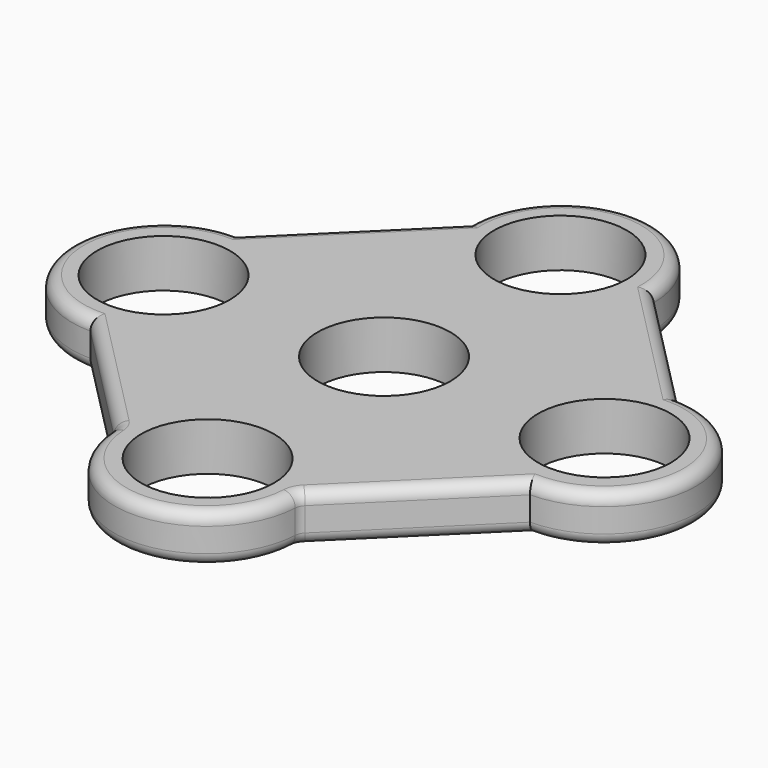
from build123d import *

# Parameters (mm, degrees)
F0_R     = 11.05
F1_DEPTH = 8
F2_R     = 2


with BuildPart() as f1:
    # F0 (on Top) → F1 (new body)
    with BuildSketch(Plane.XY):
        with BuildLine():
            Line((36.6952344775, 15.2133565883), (15.5011650662, 36.6952344775))
            ThreePointArc((15.5011650662, 36.6952344775), (0.1439042389, 52.0524953048), (-15.2133565883, 36.6952344775))
            Line((-15.2133565883, 36.6952344775), (-36.6952344775, 15.5011650662))
            ThreePointArc((-36.6952344775, 15.5011650662), (-52.0524953048, 0.1439042389), (-36.6952344775, -15.2133565883))
            Line((-36.6952344775, -15.2133565883), (-15.5011650662, -36.6952344775))
            ThreePointArc((-15.5011650662, -36.6952344775), (-0.1439042389, -52.0524953048), (15.2133565883, -36.6952344775))
            Line((15.2133565883, -36.6952344775), (36.6952344775, -15.5011650662))
            ThreePointArc((36.6952344775, -15.5011650662), (52.0524953048, -0.1439042389), (36.6952344775, 15.2133565883))
        make_face()
        with Locations((0, -36.6952344775)):
            Circle(F0_R, mode=Mode.SUBTRACT)
        with Locations((-36.6952344775, 0)):
            Circle(F0_R, mode=Mode.SUBTRACT)
        Circle(F0_R, mode=Mode.SUBTRACT)
        with Locations((0, 36.6952344775)):
            Circle(F0_R, mode=Mode.SUBTRACT)
        with Locations((36.6952344775, 0)):
            Circle(F0_R, mode=Mode.SUBTRACT)
    extrude(amount=F1_DEPTH)

    # F2
    f2_edges = [f1.edges().sort_by_distance(p)[0] for p in [
        (-25.954296, 26.0982, 8),
        (0.143904, 52.052495, 8),
        (26.0982, 25.954296, 8),
        (52.052495, -0.143904, 8),
        (25.954296, -26.0982, 8),
        (-0.143904, -52.052495, 8),
        (-26.0982, -25.954296, 8),
        (-52.052495, 0.143904, 8),
        (-15.501165, -36.695234, 4),
        (15.213357, -36.695234, 4),
        (-0.143904, -52.052495, 0),
        (25.954296, -26.0982, 0),
        (52.052495, -0.143904, 0),
        (26.0982, 25.954296, 0),
        (0.143904, 52.052495, 0),
        (-25.954296, 26.0982, 0),
        (-52.052495, 0.143904, 0),
        (-26.0982, -25.954296, 0),
    ]]
    fillet(f2_edges, radius=F2_R)


solid = f1.part
